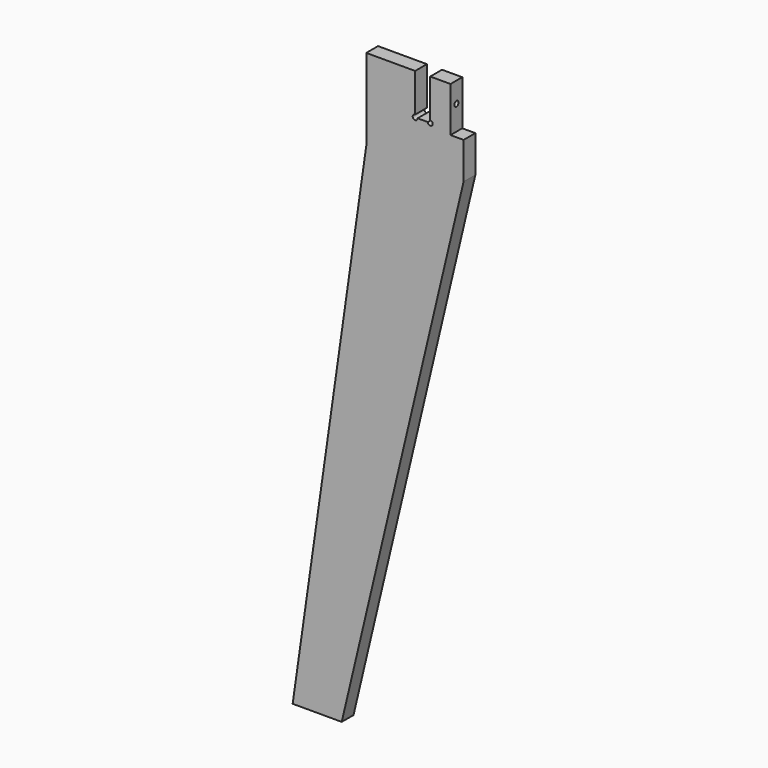
from build123d import *

# Parameters (mm, degrees)
F1_DEPTH = 18
F3_D     = 6.5
F3_DEPTH = 25
F3_TIP   = 1.9527970118


# Not quite as in the source:
# - a feature names something its author has since deleted; it is built from what else it names


with BuildPart() as f1:
    # F0 (on Front) → F1 (new body)
    with BuildSketch(Plane.XZ):
        with BuildLine():
            Line((0, 0), (0, -100))
            Line((0, -100), (-90, -730))
            Line((-90, -730), (-30, -730))
            Line((-30, -730), (119, -100))
            Line((119, -100), (119, -55))
            Line((119, -55), (103, -55))
            Line((103, -55), (103, -25))
            Line((103, -25), (103, 0))
            Line((103, 0), (78.25, 0))
            Line((78.25, 0), (78.25, -47))
            ThreePointArc((78.25, -47), (80.3713203436, -52.1213203436), (75.25, -50))
            Line((75.25, -50), (62.75, -50))
            ThreePointArc((62.75, -50), (57.6286796564, -52.1213203436), (59.75, -47))
            Line((59.75, -47), (59.75, 0))
            Line((59.75, 0), (0, 0))
        make_face()
    extrude(amount=F1_DEPTH)

    # F3
    with Locations(Plane.YZ.offset(103)):
        with Locations((-9, -25)):
            Hole(F3_D / 2, depth=F3_DEPTH)
            with Locations((0, 0, -(F3_DEPTH + F3_TIP / 2))):  # 118° drill point
                Cone(0, F3_D / 2, F3_TIP, mode=Mode.SUBTRACT)


solid = f1.part
